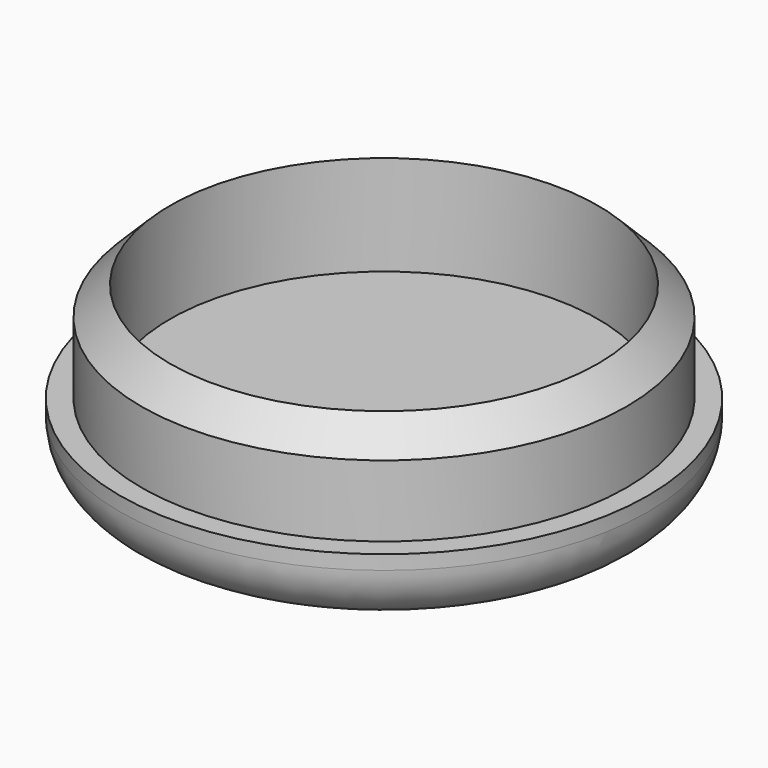
from build123d import *

# Parameters (mm, degrees)
F0_R     = 23.5061904225
F1_DEPTH = 6.35
F2_R     = 21.5857863289
F2_R_2   = 19.0486454652
F3_DEPTH = 15.24
F4_R     = 5.08


# Not quite as in the source:
# - a fillet or chamfer that OpenCascade refuses, or shapes differently, is made with other operations: its cross-section is extruded or revolved along the edge and cut away or added


with BuildPart() as f1:
    # F0 (on Top) → F1 (new body)
    with BuildSketch(Plane.XY):
        Circle(F0_R)
    extrude(amount=F1_DEPTH)

    # F2 (on Top) → F3 (join)
    with BuildSketch(Plane.XY):
        Circle(F2_R)
        Circle(F2_R_2, mode=Mode.SUBTRACT)
    extrude(amount=F3_DEPTH)

    # F4
    f4_edges = [f1.edges().sort_by_distance(p)[0] for p in [
        (-23.50619, 0, 0),
    ]]
    fillet(f4_edges, radius=F4_R)

    # F5: chamfer of 2.54 on 1 edges, made by hand

    # F5_s1 → F5_t2 (revolve, cut)
    with BuildSketch(Plane.XZ):
        Polygon((21.5857863289, 12.7), (19.0457863289, 15.24), (21.5857863289, 15.24), align=None)
    revolve(axis=Axis((0, 0, 15.24), (0, 0, 1)), mode=Mode.SUBTRACT)


solid = f1.part
